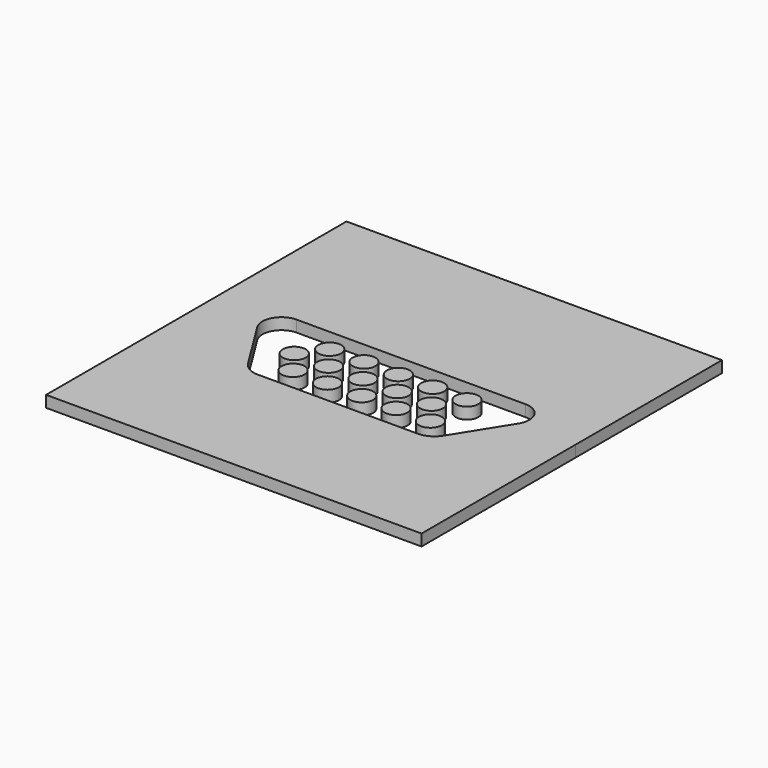
from build123d import *

# Parameters (mm, degrees)
F0_R     = 1
F1_DEPTH = 1
F2_DEPTH = 1


# Not quite as in the source:
# - ends of sketch curves that miss each other by under 0.0002 mm in the source are joined


with BuildPart() as f1:
    # F0 (on Top) → F1 (new body)
    with BuildSketch(Plane.XY):
        with Locations((-4.5, 2)):
            Circle(F0_R)
    extrude(amount=F1_DEPTH)


with BuildPart() as f1b:
    # F0 (on Top) → F1, piece 2 (new body)
    with BuildSketch(Plane.XY):
        with Locations((-1.5, 2)):
            Circle(F0_R)
    extrude(amount=F1_DEPTH)


with BuildPart() as f1c:
    # F0 (on Top) → F1, piece 3 (new body)
    with BuildSketch(Plane.XY):
        with Locations((1.5, 2)):
            Circle(F0_R)
    extrude(amount=F1_DEPTH)


with BuildPart() as f1d:
    # F0 (on Top) → F1, piece 4 (new body)
    with BuildSketch(Plane.XY):
        with Locations((4.5, 2)):
            Circle(F0_R)
    extrude(amount=F1_DEPTH)


with BuildPart() as f1e:
    # F0 (on Top) → F1, piece 5 (new body)
    with BuildSketch(Plane.XY):
        with Locations((7.5, 2)):
            Circle(F0_R)
    extrude(amount=F1_DEPTH)


with BuildPart() as f1f:
    # F0 (on Top) → F1, piece 6 (new body)
    with BuildSketch(Plane.XY):
        with Locations((6, 0)):
            Circle(F0_R)
    extrude(amount=F1_DEPTH)


with BuildPart() as f1g:
    # F0 (on Top) → F1, piece 7 (new body)
    with BuildSketch(Plane.XY):
        with Locations((3, 0)):
            Circle(F0_R)
    extrude(amount=F1_DEPTH)


with BuildPart() as f1h:
    # F0 (on Top) → F1, piece 8 (new body)
    with BuildSketch(Plane.XY):
        Circle(F0_R)
    extrude(amount=F1_DEPTH)


with BuildPart() as f1i:
    # F0 (on Top) → F1, piece 9 (new body)
    with BuildSketch(Plane.XY):
        with Locations((-3, 0)):
            Circle(F0_R)
    extrude(amount=F1_DEPTH)


with BuildPart() as f1j:
    # F0 (on Top) → F1, piece 10 (new body)
    with BuildSketch(Plane.XY):
        with Locations((-6, 0)):
            Circle(F0_R)
    extrude(amount=F1_DEPTH)


with BuildPart() as f1k:
    # F0 (on Top) → F1, piece 11 (new body)
    with BuildSketch(Plane.XY):
        with Locations((-4.5, -2)):
            Circle(F0_R)
    extrude(amount=F1_DEPTH)


with BuildPart() as f1l:
    # F0 (on Top) → F1, piece 12 (new body)
    with BuildSketch(Plane.XY):
        with Locations((-1.5, -2)):
            Circle(F0_R)
    extrude(amount=F1_DEPTH)


with BuildPart() as f1m:
    # F0 (on Top) → F1, piece 13 (new body)
    with BuildSketch(Plane.XY):
        with Locations((1.5, -2)):
            Circle(F0_R)
    extrude(amount=F1_DEPTH)


with BuildPart() as f1n:
    # F0 (on Top) → F1, piece 14 (new body)
    with BuildSketch(Plane.XY):
        with Locations((4.5, -2)):
            Circle(F0_R)
    extrude(amount=F1_DEPTH)


with BuildPart() as f1o:
    # F0 (on Top) → F1, piece 15 (new body)
    with BuildSketch(Plane.XY):
        with Locations((7.5, -2)):
            Circle(F0_R)
    extrude(amount=F1_DEPTH)


with BuildPart() as f2:
    # F0 (on Top) → F2 (new body)
    with BuildSketch(Plane.XY):
        Polygon((17.4168121663, -15.363994912), (17.4168121663, 1.456005088), (17.4168185263, 17.456005088), (-15.4031878337, 17.456005088), (-15.4031878337, -15.363994912), align=None)
        with BuildLine():
            Line((-8.9931846537, 4), (0.0068153463, 4))
            Line((0.0068153463, 4), (11.0068153463, 4))
            ThreePointArc((11.0068153463, 4), (12.4611209434, 3.1433025227), (12.4168185263, 1.456005088))
            Line((12.4168185263, 1.456005088), (9.5368142863, -3.152001696))
            ThreePointArc((9.5368142863, -3.152001696), (8.8814578275, -3.7738239924), (8.0068153463, -4))
            Line((8.0068153463, -4), (-5.9931846537, -4))
            ThreePointArc((-5.9931846537, -4), (-6.867827135, -3.7738239924), (-7.5231835937, -3.152001696))
            Line((-7.5231835937, -3.152001696), (-10.4031878337, 1.456005088))
            ThreePointArc((-10.4031878337, 1.456005088), (-10.4474902509, 3.1433025227), (-8.9931846537, 4))
        make_face(mode=Mode.SUBTRACT)
    extrude(amount=F2_DEPTH)


solid = Compound([f1.part, f1b.part, f1c.part, f1d.part, f1e.part, f1f.part, f1g.part, f1h.part, f1i.part, f1j.part, f1k.part, f1l.part, f1m.part, f1n.part, f1o.part, f2.part])
